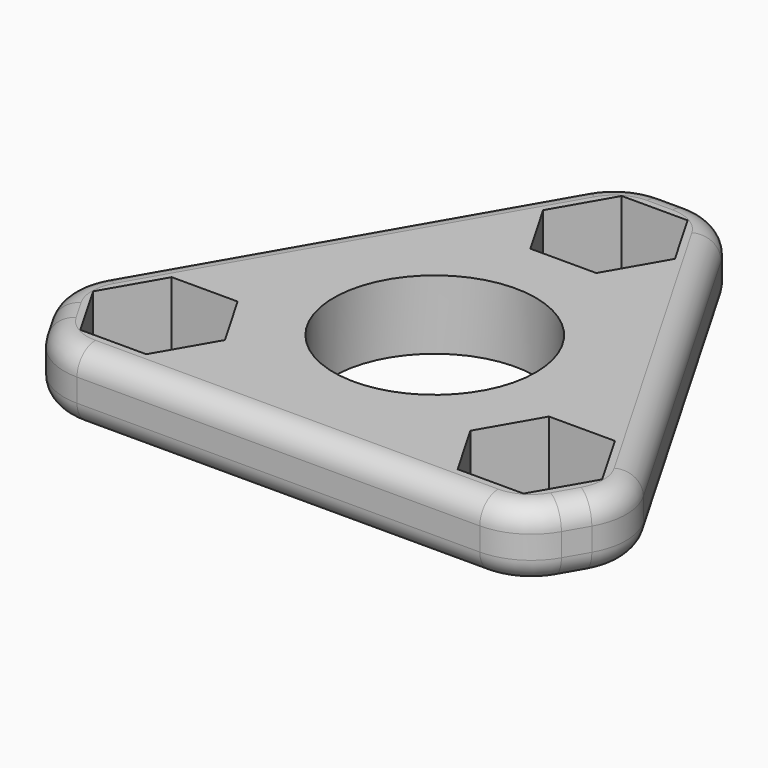
from build123d import *

# Parameters (mm, degrees)
F0_R     = 10.975
F1_DEPTH = 3.75
F2_R     = 7
F3_R     = 2.5


# Not quite as in the source:
# - a feature names something its author has since deleted; it is built from what else it names


with BuildPart() as f1:
    # F0 (on Top) → F1 (new body, symmetric)
    with BuildSketch(Plane.XY):
        Polygon((-5.4270925304, 33.057475201), (-10.8541850608, 23.657475201), (-25.9150670439, -2.4287376005), (-31.3421595743, -11.8287376005), (-25.9150670439, -21.2287376005), (-15.0608819831, -21.2287376005), (15.0608819831, -21.2287376005), (25.9150670439, -21.2287376005), (31.3421595743, -11.8287376005), (25.9150670439, -2.4287376005), (10.8541850608, 23.657475201), (5.4270925304, 33.057475201), align=None)
        Polygon((-16.9084028445, -5.6287376005), (-13.3288311755, -11.8287376005), (-16.9084028445, -18.0287376005), (-24.0675461825, -18.0287376005), (-27.6471178514, -11.8287376005), (-24.0675461825, -5.6287376005), align=None, mode=Mode.SUBTRACT)
        Circle(F0_R, mode=Mode.SUBTRACT)
        Polygon((24.0675461825, -5.6287376005), (27.6471178514, -11.8287376005), (24.0675461825, -18.0287376005), (16.9084028445, -18.0287376005), (13.3288311755, -11.8287376005), (16.9084028445, -5.6287376005), align=None, mode=Mode.SUBTRACT)
        Polygon((3.579571669, 29.857475201), (7.159143338, 23.657475201), (3.579571669, 17.457475201), (-3.579571669, 17.457475201), (-7.159143338, 23.657475201), (-3.579571669, 29.857475201), align=None, mode=Mode.SUBTRACT)
    extrude(amount=F1_DEPTH, both=True)

    # F2
    f2_edges = [f1.edges().sort_by_distance(p)[0] for p in [
        (31.34216, -11.828738, 0),
        (25.915067, -21.228738, 0),
        (-25.915067, -21.228738, 0),
        (-31.34216, -11.828738, 0),
        (-5.427093, 33.057475, 0),
        (5.427093, 33.057475, 0),
    ]]
    fillet(f2_edges, radius=F2_R)

    # F3
    f3_edges = [f1.edges().sort_by_distance(p)[0] for p in [
        (-18.384626, 10.614369, -3.75),
        (-7.447818, 29.557475, 0),
        (-29.321434, -8.328738, 0),
        (-18.384626, 10.614369, 3.75),
    ]]
    fillet(f3_edges, radius=F3_R)


solid = f1.part
